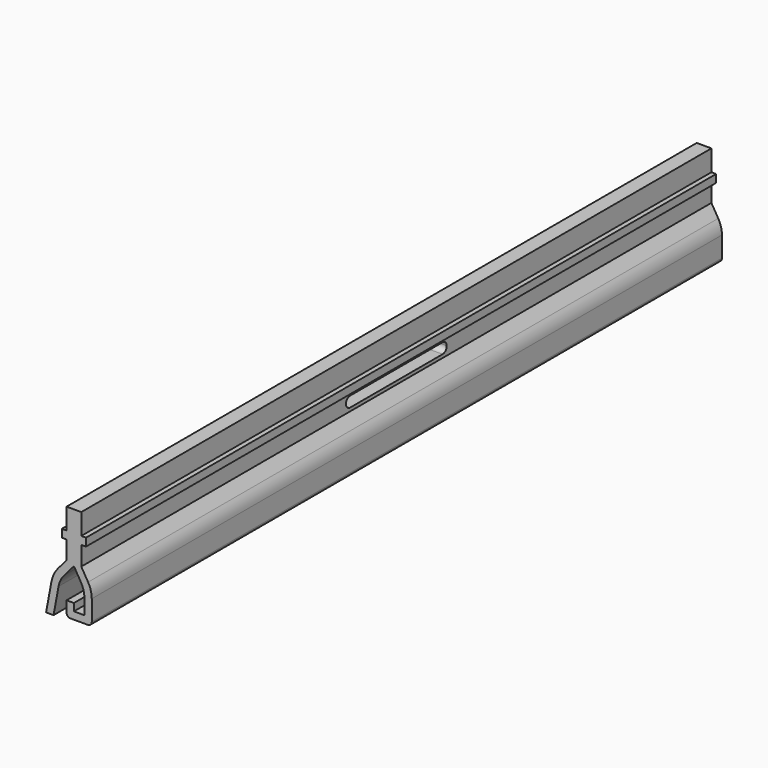
from build123d import *

# Parameters (mm, degrees)
F1_DEPTH = 75
F3_DEPTH = 12.5


# Not quite as in the source:
# - ends of sketch curves that miss each other by under 0.0002 mm in the source are joined


with BuildPart() as f1:
    # F0 (on Front) → F1 (new body, symmetric)
    with BuildSketch(Plane.XZ):
        with BuildLine():
            Line((1.4, 9), (-1.4, 9))
            Line((-1.4, 9), (-1.4, 5))
            Line((-1.4, 5), (-2.3, 5))
            Line((-2.3, 5), (-2.3, 3.5))
            Line((-2.3, 3.5), (-1.4, 3.5))
            Line((-1.4, 3.5), (-1.4, 0))
            Line((-1.4, 0), (-2.932592, -1.768375))
            ThreePointArc((-2.932592, -1.768375), (-3.80412, -3.094345), (-4.297589, -4.602405))
            Line((-4.297589, -4.602405), (-5.3, -10))
            Line((-5.3, -10), (-3.876062, -10))
            Line((-3.876062, -10), (-2.921314, -4.859053))
            ThreePointArc((-2.921314, -4.859053), (-2.543024, -3.702321), (-1.874627, -2.685278))
            Line((-1.874627, -2.685278), (0, -0.522247))
            Line((0, -0.522247), (1.297343, -2.703488))
            ThreePointArc((1.297343, -2.703488), (1.821137, -3.934047), (2, -5.259431))
            Line((2, -5.259431), (2, -8.1))
            Line((2, -8.1), (0, -8.1))
            Line((0, -8.1), (0, -6.7))
            Line((0, -6.7), (-1.4, -6.7))
            Line((-1.4, -6.7), (-1.4, -8.75))
            ThreePointArc((-1.4, -8.75), (-1.18033, -9.28033), (-0.65, -9.5))
            Line((-0.65, -9.5), (2.65, -9.5))
            ThreePointArc((2.65, -9.5), (3.18033, -9.28033), (3.4, -8.75))
            Line((3.4, -8.75), (3.4, -4.874555))
            ThreePointArc((3.4, -4.874555), (3.221137, -3.549172), (2.697343, -2.318613))
            Line((2.697343, -2.318613), (1.4, -0.137371))
            Line((1.4, -0.137371), (1.4, 3.5))
            Line((1.4, 3.5), (2.3, 3.5))
            Line((2.3, 3.5), (2.3, 5))
            Line((2.3, 5), (1.4, 5))
            Line((1.4, 5), (1.4, 9))
        make_face()
    extrude(amount=F1_DEPTH, both=True)

    # F2 (on Right) → F3 (cut, symmetric)
    with BuildSketch(Plane.YZ):
        with BuildLine():
            ThreePointArc((12, 1.5), (11.707107, 2.207107), (11, 2.5))
            Line((11, 2.5), (-11, 2.5))
            ThreePointArc((-11, 2.5), (-11.707107, 2.207107), (-12, 1.5))
            ThreePointArc((-12, 1.5), (-11.707107, 0.792893), (-11, 0.5))
            Line((-11, 0.5), (11, 0.5))
            ThreePointArc((11, 0.5), (11.707107, 0.792893), (12, 1.5))
        make_face()
    extrude(amount=F3_DEPTH, both=True, mode=Mode.SUBTRACT)


solid = f1.part
